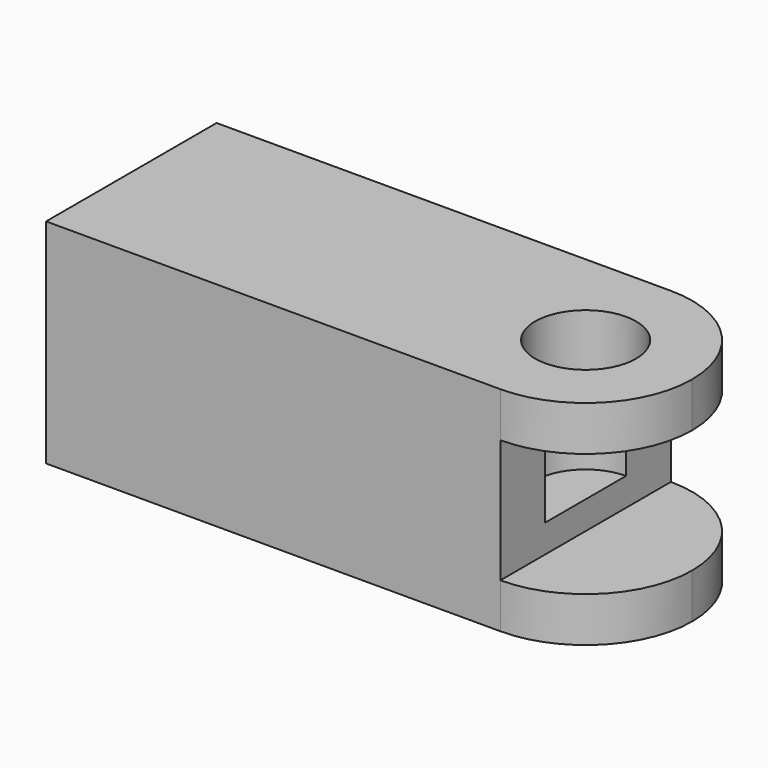
from build123d import *

# Parameters (mm, degrees)
F0_W     = 100
F0_H     = 38
F1_DEPTH = 38
F2_R     = 18.99999
F3_R     = 9
F4_DEPTH = 25
F5_W     = 20.3221625665
F5_H     = 22
F6_DEPTH = 38.001


# Not quite as in the source:
# - a fillet or chamfer is up to 0.001 mm smaller than in the source, because OpenCascade refuses the exact size


with BuildPart() as f1:
    # F0 (on Top) → F1 (new body)
    with BuildSketch(Plane.XY):
        with Locations((50, 19)):
            Rectangle(F0_W, F0_H)
    extrude(amount=F1_DEPTH)

    # F2 (radius 19 in the source; OpenCascade refuses exactly that, so slightly less here)
    f2_edges = [f1.edges().sort_by_distance(p)[0] for p in [
        (100, 0, 19),
        (100, 38, 19),
    ]]
    fillet(f2_edges, radius=F2_R)

    # F3 (on face) → F4 (cut)
    with BuildSketch(Plane.XY.offset(38)):
        with Locations((81, 19)):
            Circle(F3_R)
    extrude(amount=-F4_DEPTH, mode=Mode.SUBTRACT)

    # F5 (on face) → F6 (cut, through all)
    with BuildSketch(Plane.XZ):
        with Locations((91.1610912833, 19)):
            Rectangle(F5_W, F5_H)
    extrude(amount=-F6_DEPTH, mode=Mode.SUBTRACT)


solid = f1.part
